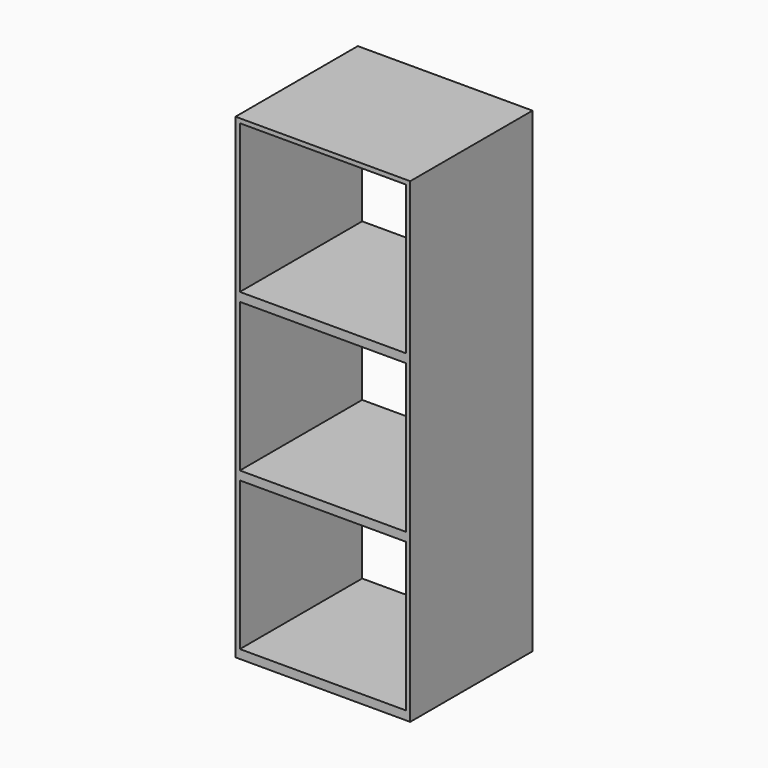
from build123d import *

# Parameters (mm, degrees)
F0_W     = 400
F0_H     = 350
F1_DEPTH = 1600
F2_W     = 190
F2_H     = 340
F3_DEPTH = 350
F4_DEPTH = 500
F5_DEPTH = 10


# Not quite as in the source:
# - a feature names something its author has since deleted; it is built from what else it names


with BuildPart() as f1:
    # F0 (on Top) → F1 (new body)
    with BuildSketch(Plane.XY):
        with Locations((200, 175)):
            Rectangle(F0_W, F0_H)
    extrude(amount=F1_DEPTH)

    # F2 (on face) → F3 (cut)
    with BuildSketch(Plane.XZ):
        with Locations((295, 1420)):
            Rectangle(F2_W, F2_H)
        with Locations((105, 1420)):
            Rectangle(F2_W, F2_H)
        with Locations((105, 1060)):
            Rectangle(F2_W, F2_H)
        with Locations((295, 1060)):
            Rectangle(F2_W, F2_H)
        with Locations((295, 700)):
            Rectangle(F2_W, F2_H)
        with Locations((105, 700)):
            Rectangle(F2_W, F2_H)
    extrude(amount=-F3_DEPTH, mode=Mode.SUBTRACT)

    # F4 (cut): a face of the model
    f4_faces = [f1.faces().sort_by_distance(p)[0] for p in [
        (200, 175, 0),
    ]]
    extrude(f4_faces, amount=-F4_DEPTH, mode=Mode.SUBTRACT)

    # F5 (cut): a face of the model
    f5_faces = [f1.faces().sort_by_distance(p)[0] for p in [
        (200, 175, 500),
    ]]
    extrude(f5_faces, amount=-F5_DEPTH, mode=Mode.SUBTRACT)


solid = f1.part
